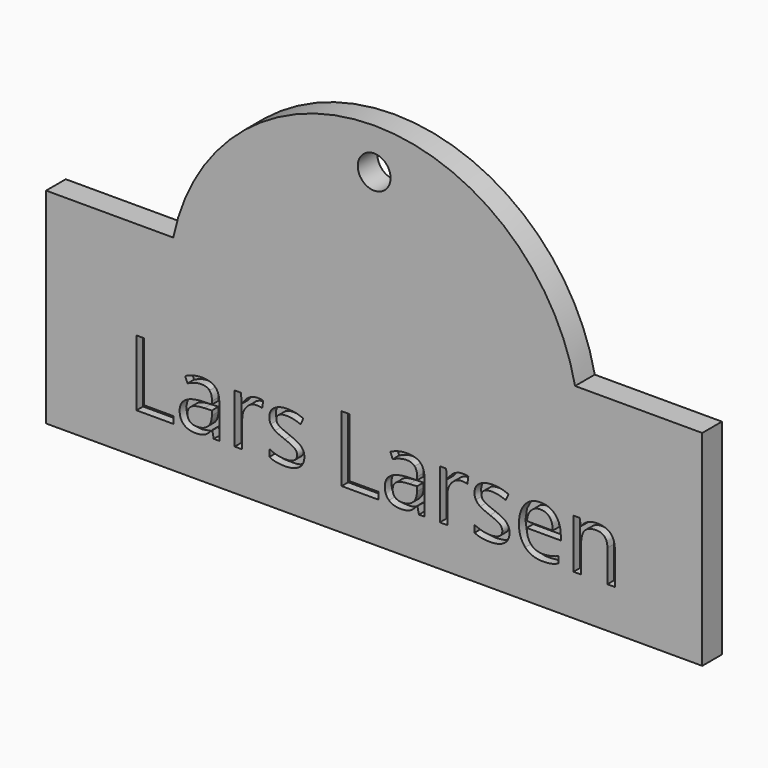
from build123d import *

# Parameters (mm, degrees)
F0_R         = 2
F1_DEPTH     = 3
F0_TEXT_SIZE = 11.2661289879
F2_DEPTH     = 2


# Not quite as in the source:
# - Text() gives the source's letters only with a copy of the font that has no kerning and outlines rounded to 1/6400 em; it was checked with that copy


with BuildPart() as f1:
    # F0 (on Front) → F1 (new body)
    with BuildSketch(Plane.XZ):
        with BuildLine():
            Line((-80.8457088497, 41.3709692657), (-96.3508114219, 41.3709692657))
            Line((-96.3508114219, 41.3709692657), (-96.3508114219, 16.3709692657))
            Line((-96.3508114219, 16.3709692657), (-16.3508114219, 16.3709692657))
            Line((-16.3508114219, 16.3709692657), (-16.3508114219, 41.3709692657))
            Line((-16.3508114219, 41.3709692657), (-31.855913994, 41.3709692657))
            ThreePointArc((-31.855913994, 41.3709692657), (-56.3508114219, 61.3709692657), (-80.8457088497, 41.3709692657))
        make_face()
        with BuildLine():
            Line((-75.2303791399, 21.3709692657), (-75.9081072118, 21.3709692657))
            Line((-75.9081072118, 21.3709692657), (-76.0894214752, 22.230011601))
            Line((-76.0894214752, 22.230011601), (-76.1334297916, 22.230011601))
            add(Edge.make_bspline(
                [(-76.1334297916, 22.230011601), (-76.5840749511, 21.6631844863), (-77.0320796116, 21.4616263974)],
                knots=[0, 0, 0, 1, 1, 1], degree=2))
            add(Edge.make_bspline(
                [(-77.0320796116, 21.4616263974), (-77.4800842721, 21.2600683085), (-78.1525313461, 21.2600683085)],
                knots=[0, 0, 0, 1, 1, 1], degree=2))
            add(Edge.make_bspline(
                [(-78.1525313461, 21.2600683085), (-79.0485406672, 21.2600683085), (-79.5572768043, 21.7230357966)],
                knots=[0, 0, 0, 1, 1, 1], degree=2))
            add(Edge.make_bspline(
                [(-79.5572768043, 21.7230357966), (-80.0660129414, 22.1860032847), (-80.0660129414, 23.0380042894)],
                knots=[0, 0, 0, 1, 1, 1], degree=2))
            add(Edge.make_bspline(
                [(-80.0660129414, 23.0380042894), (-80.0660129414, 24.8634692519), (-77.1456210678, 24.9514858847)],
                knots=[0, 0, 0, 1, 1, 1], degree=2))
            Line((-77.1456210678, 24.9514858847), (-76.1228677956, 24.9849322051))
            Line((-76.1228677956, 24.9849322051), (-76.1228677956, 25.3598830605))
            add(Edge.make_bspline(
                [(-76.1228677956, 25.3598830605), (-76.1228677956, 26.0692971202), (-76.4274053448, 26.4072809898)],
                knots=[0, 0, 0, 1, 1, 1], degree=2))
            add(Edge.make_bspline(
                [(-76.4274053448, 26.4072809898), (-76.731942894, 26.7452648595), (-77.404389968, 26.7452648595)],
                knots=[0, 0, 0, 1, 1, 1], degree=2))
            add(Edge.make_bspline(
                [(-77.404389968, 26.7452648595), (-78.1578123441, 26.7452648595), (-79.1083919774, 26.284057704)],
                knots=[0, 0, 0, 1, 1, 1], degree=2))
            Line((-79.1083919774, 26.284057704), (-79.3900452021, 26.9829097678))
            add(Edge.make_bspline(
                [(-79.3900452021, 26.9829097678), (-78.9446810406, 27.2240753414), (-78.4139407453, 27.3613812885)],
                knots=[0, 0, 0, 1, 1, 1], degree=2))
            add(Edge.make_bspline(
                [(-78.4139407453, 27.3613812885), (-77.88320045, 27.4986872355), (-77.3480593231, 27.4986872355)],
                knots=[0, 0, 0, 1, 1, 1], degree=2))
            add(Edge.make_bspline(
                [(-77.3480593231, 27.4986872355), (-76.2707357386, 27.4986872355), (-75.7505574392, 27.0207569199)],
                knots=[0, 0, 0, 1, 1, 1], degree=2))
            add(Edge.make_bspline(
                [(-75.7505574392, 27.0207569199), (-75.2303791399, 26.5428266042), (-75.2303791399, 25.4866270116)],
                knots=[0, 0, 0, 1, 1, 1], degree=2))
            Line((-75.2303791399, 25.4866270116), (-75.2303791399, 21.3709692657))
        make_face(mode=Mode.SUBTRACT)
        Polygon((-80.842319642, 21.3709692657), (-85.3258869126, 21.3709692657), (-85.3258869126, 29.4139291635), (-84.3911502732, 29.4139291635), (-84.3911502732, 22.2176892724), (-80.842319642, 22.2176892724), align=None, mode=Mode.SUBTRACT)
        with BuildLine():
            add(Edge.make_bspline(
                [(-71.639300525, 27.1915091873), (-71.165771041, 27.5110095641), (-70.5989439263, 27.5110095641)],
                knots=[0, 0, 0, 1, 1, 1], degree=2))
            add(Edge.make_bspline(
                [(-70.5989439263, 27.5110095641), (-70.1975880811, 27.5110095641), (-69.8789678706, 27.4441169232)],
                knots=[0, 0, 0, 1, 1, 1], degree=2))
            Line((-69.8789678706, 27.4441169232), (-70.0057118217, 26.5973969165))
            add(Edge.make_bspline(
                [(-70.0057118217, 26.5973969165), (-70.3789023445, 26.6801325512), (-70.6658365671, 26.6801325512)],
                knots=[0, 0, 0, 1, 1, 1], degree=2))
            add(Edge.make_bspline(
                [(-70.6658365671, 26.6801325512), (-71.3981349513, 26.6801325512), (-71.9174330844, 26.0860202804)],
                knots=[0, 0, 0, 1, 1, 1], degree=2))
            add(Edge.make_bspline(
                [(-71.9174330844, 26.0860202804), (-72.4367312174, 25.4919080096), (-72.4367312174, 24.6064606844)],
                knots=[0, 0, 0, 1, 1, 1], degree=2))
            Line((-72.4367312174, 24.6064606844), (-72.4367312174, 21.3709692657))
            Line((-72.4367312174, 21.3709692657), (-73.350343865, 21.3709692657))
            Line((-73.350343865, 21.3709692657), (-73.350343865, 27.4001086069))
            Line((-73.350343865, 27.4001086069), (-72.596921489, 27.4001086069))
            Line((-72.596921489, 27.4001086069), (-72.4913015297, 26.284057704))
            Line((-72.4913015297, 26.284057704), (-72.4472932133, 26.284057704))
            add(Edge.make_bspline(
                [(-72.4472932133, 26.284057704), (-72.112830009, 26.8720088106), (-71.639300525, 27.1915091873)],
                knots=[0, 0, 0, 1, 1, 1], degree=2))
        make_face(mode=Mode.SUBTRACT)
        with BuildLine():
            add(Edge.make_bspline(
                [(-65.2387309937, 24.0114682472), (-64.8620198057, 23.6153934), (-64.8620198057, 23.0151199649)],
                knots=[0, 0, 0, 1, 1, 1], degree=2))
            add(Edge.make_bspline(
                [(-64.8620198057, 23.0151199649), (-64.8620198057, 22.1736809561), (-65.4886982307, 21.7168746323)],
                knots=[0, 0, 0, 1, 1, 1], degree=2))
            add(Edge.make_bspline(
                [(-65.4886982307, 21.7168746323), (-66.1153766556, 21.2600683085), (-67.249030885, 21.2600683085)],
                knots=[0, 0, 0, 1, 1, 1], degree=2))
            add(Edge.make_bspline(
                [(-67.249030885, 21.2600683085), (-68.4478174226, 21.2600683085), (-69.1185041639, 21.6403001618)],
                knots=[0, 0, 0, 1, 1, 1], degree=2))
            Line((-69.1185041639, 21.6403001618), (-69.1185041639, 22.4870201686))
            add(Edge.make_bspline(
                [(-69.1185041639, 22.4870201686), (-68.6837019983, 22.2669785868), (-68.1864080235, 22.141114802)],
                knots=[0, 0, 0, 1, 1, 1], degree=2))
            add(Edge.make_bspline(
                [(-68.1864080235, 22.141114802), (-67.6891140486, 22.0152510172), (-67.2261465605, 22.0152510172)],
                knots=[0, 0, 0, 1, 1, 1], degree=2))
            add(Edge.make_bspline(
                [(-67.2261465605, 22.0152510172), (-66.5114515028, 22.0152510172), (-66.1268188179, 22.2432140959)],
                knots=[0, 0, 0, 1, 1, 1], degree=2))
            add(Edge.make_bspline(
                [(-66.1268188179, 22.2432140959), (-65.7421861329, 22.4711771747), (-65.7421861329, 22.9394256607)],
                knots=[0, 0, 0, 1, 1, 1], degree=2))
            add(Edge.make_bspline(
                [(-65.7421861329, 22.9394256607), (-65.7421861329, 23.2914921916), (-66.0467236821, 23.5414594285)],
                knots=[0, 0, 0, 1, 1, 1], degree=2))
            add(Edge.make_bspline(
                [(-66.0467236821, 23.5414594285), (-66.3512612313, 23.7914266654), (-67.2384688891, 24.1329312004)],
                knots=[0, 0, 0, 1, 1, 1], degree=2))
            add(Edge.make_bspline(
                [(-67.2384688891, 24.1329312004), (-68.0799078979, 24.4462704129), (-68.4346149277, 24.6803946559)],
                knots=[0, 0, 0, 1, 1, 1], degree=2))
            add(Edge.make_bspline(
                [(-68.4346149277, 24.6803946559), (-68.7893219576, 24.9145188989), (-68.962714724, 25.2111349512)],
                knots=[0, 0, 0, 1, 1, 1], degree=2))
            add(Edge.make_bspline(
                [(-68.962714724, 25.2111349512), (-69.1361074905, 25.5077510034), (-69.1361074905, 25.9196688446)],
                knots=[0, 0, 0, 1, 1, 1], degree=2))
            add(Edge.make_bspline(
                [(-69.1361074905, 25.9196688446), (-69.1361074905, 26.6572482267), (-68.5358340553, 27.0841288954)],
                knots=[0, 0, 0, 1, 1, 1], degree=2))
            add(Edge.make_bspline(
                [(-68.5358340553, 27.0841288954), (-67.9355606202, 27.5110095641), (-66.8916833562, 27.5110095641)],
                knots=[0, 0, 0, 1, 1, 1], degree=2))
            add(Edge.make_bspline(
                [(-66.8916833562, 27.5110095641), (-65.9182193983, 27.5110095641), (-64.9870034242, 27.1149347169)],
                knots=[0, 0, 0, 1, 1, 1], degree=2))
            Line((-64.9870034242, 27.1149347169), (-65.3126649652, 26.3720743367))
            add(Edge.make_bspline(
                [(-65.3126649652, 26.3720743367), (-66.2192362822, 26.7452648595), (-66.9568156644, 26.7452648595)],
                knots=[0, 0, 0, 1, 1, 1], degree=2))
            add(Edge.make_bspline(
                [(-66.9568156644, 26.7452648595), (-67.6063784138, 26.7452648595), (-67.9364407865, 26.5419464379)],
                knots=[0, 0, 0, 1, 1, 1], degree=2))
            add(Edge.make_bspline(
                [(-67.9364407865, 26.5419464379), (-68.2665031592, 26.3386280163), (-68.2665031592, 25.9812804875)],
                knots=[0, 0, 0, 1, 1, 1], degree=2))
            add(Edge.make_bspline(
                [(-68.2665031592, 25.9812804875), (-68.2665031592, 25.7383545812), (-68.1423997071, 25.56848248)],
                knots=[0, 0, 0, 1, 1, 1], degree=2))
            add(Edge.make_bspline(
                [(-68.1423997071, 25.56848248), (-68.018296255, 25.3986103789), (-67.7436843609, 25.2445812716)],
                knots=[0, 0, 0, 1, 1, 1], degree=2))
            add(Edge.make_bspline(
                [(-67.7436843609, 25.2445812716), (-67.4690724668, 25.0905521644), (-66.6874847683, 24.7983369437)],
                knots=[0, 0, 0, 1, 1, 1], degree=2))
            add(Edge.make_bspline(
                [(-66.6874847683, 24.7983369437), (-65.6154421818, 24.4075430945), (-65.2387309937, 24.0114682472)],
                knots=[0, 0, 0, 1, 1, 1], degree=2))
        make_face(mode=Mode.SUBTRACT)
        Polygon((-55.8279926235, 21.3709692657), (-60.3115598942, 21.3709692657), (-60.3115598942, 29.4139291635), (-59.3768232547, 29.4139291635), (-59.3768232547, 22.2176892724), (-55.8279926235, 22.2176892724), align=None, mode=Mode.SUBTRACT)
        with BuildLine():
            Line((-50.2160521214, 21.3709692657), (-50.8937801934, 21.3709692657))
            Line((-50.8937801934, 21.3709692657), (-51.0750944568, 22.230011601))
            Line((-51.0750944568, 22.230011601), (-51.1191027731, 22.230011601))
            add(Edge.make_bspline(
                [(-51.1191027731, 22.230011601), (-51.5697479326, 21.6631844863), (-52.0177525932, 21.4616263974)],
                knots=[0, 0, 0, 1, 1, 1], degree=2))
            add(Edge.make_bspline(
                [(-52.0177525932, 21.4616263974), (-52.4657572537, 21.2600683085), (-53.1382043277, 21.2600683085)],
                knots=[0, 0, 0, 1, 1, 1], degree=2))
            add(Edge.make_bspline(
                [(-53.1382043277, 21.2600683085), (-54.0342136487, 21.2600683085), (-54.5429497858, 21.7230357966)],
                knots=[0, 0, 0, 1, 1, 1], degree=2))
            add(Edge.make_bspline(
                [(-54.5429497858, 21.7230357966), (-55.051685923, 22.1860032847), (-55.051685923, 23.0380042894)],
                knots=[0, 0, 0, 1, 1, 1], degree=2))
            add(Edge.make_bspline(
                [(-55.051685923, 23.0380042894), (-55.051685923, 24.8634692519), (-52.1312940494, 24.9514858847)],
                knots=[0, 0, 0, 1, 1, 1], degree=2))
            Line((-52.1312940494, 24.9514858847), (-51.1085407772, 24.9849322051))
            Line((-51.1085407772, 24.9849322051), (-51.1085407772, 25.3598830605))
            add(Edge.make_bspline(
                [(-51.1085407772, 25.3598830605), (-51.1085407772, 26.0692971202), (-51.4130783264, 26.4072809898)],
                knots=[0, 0, 0, 1, 1, 1], degree=2))
            add(Edge.make_bspline(
                [(-51.4130783264, 26.4072809898), (-51.7176158756, 26.7452648595), (-52.3900629496, 26.7452648595)],
                knots=[0, 0, 0, 1, 1, 1], degree=2))
            add(Edge.make_bspline(
                [(-52.3900629496, 26.7452648595), (-53.1434853256, 26.7452648595), (-54.094064959, 26.284057704)],
                knots=[0, 0, 0, 1, 1, 1], degree=2))
            Line((-54.094064959, 26.284057704), (-54.3757181837, 26.9829097678))
            add(Edge.make_bspline(
                [(-54.3757181837, 26.9829097678), (-53.9303540221, 27.2240753414), (-53.3996137268, 27.3613812885)],
                knots=[0, 0, 0, 1, 1, 1], degree=2))
            add(Edge.make_bspline(
                [(-53.3996137268, 27.3613812885), (-52.8688734315, 27.4986872355), (-52.3337323046, 27.4986872355)],
                knots=[0, 0, 0, 1, 1, 1], degree=2))
            add(Edge.make_bspline(
                [(-52.3337323046, 27.4986872355), (-51.2564087202, 27.4986872355), (-50.7362304208, 27.0207569199)],
                knots=[0, 0, 0, 1, 1, 1], degree=2))
            add(Edge.make_bspline(
                [(-50.7362304208, 27.0207569199), (-50.2160521214, 26.5428266042), (-50.2160521214, 25.4866270116)],
                knots=[0, 0, 0, 1, 1, 1], degree=2))
            Line((-50.2160521214, 25.4866270116), (-50.2160521214, 21.3709692657))
        make_face(mode=Mode.SUBTRACT)
        with BuildLine():
            add(Edge.make_bspline(
                [(-46.6249735065, 27.1915091873), (-46.1514440225, 27.5110095641), (-45.5846169078, 27.5110095641)],
                knots=[0, 0, 0, 1, 1, 1], degree=2))
            add(Edge.make_bspline(
                [(-45.5846169078, 27.5110095641), (-45.1832610626, 27.5110095641), (-44.8646408522, 27.4441169232)],
                knots=[0, 0, 0, 1, 1, 1], degree=2))
            Line((-44.8646408522, 27.4441169232), (-44.9913848033, 26.5973969165))
            add(Edge.make_bspline(
                [(-44.9913848033, 26.5973969165), (-45.364575326, 26.6801325512), (-45.6515095487, 26.6801325512)],
                knots=[0, 0, 0, 1, 1, 1], degree=2))
            add(Edge.make_bspline(
                [(-45.6515095487, 26.6801325512), (-46.3838079329, 26.6801325512), (-46.9031060659, 26.0860202804)],
                knots=[0, 0, 0, 1, 1, 1], degree=2))
            add(Edge.make_bspline(
                [(-46.9031060659, 26.0860202804), (-47.422404199, 25.4919080096), (-47.422404199, 24.6064606844)],
                knots=[0, 0, 0, 1, 1, 1], degree=2))
            Line((-47.422404199, 24.6064606844), (-47.422404199, 21.3709692657))
            Line((-47.422404199, 21.3709692657), (-48.3360168466, 21.3709692657))
            Line((-48.3360168466, 21.3709692657), (-48.3360168466, 27.4001086069))
            Line((-48.3360168466, 27.4001086069), (-47.5825944705, 27.4001086069))
            Line((-47.5825944705, 27.4001086069), (-47.4769745112, 26.284057704))
            Line((-47.4769745112, 26.284057704), (-47.4329661949, 26.284057704))
            add(Edge.make_bspline(
                [(-47.4329661949, 26.284057704), (-47.0985029906, 26.8720088106), (-46.6249735065, 27.1915091873)],
                knots=[0, 0, 0, 1, 1, 1], degree=2))
        make_face(mode=Mode.SUBTRACT)
        with BuildLine():
            add(Edge.make_bspline(
                [(-40.2244039753, 24.0114682472), (-39.8476927872, 23.6153934), (-39.8476927872, 23.0151199649)],
                knots=[0, 0, 0, 1, 1, 1], degree=2))
            add(Edge.make_bspline(
                [(-39.8476927872, 23.0151199649), (-39.8476927872, 22.1736809561), (-40.4743712122, 21.7168746323)],
                knots=[0, 0, 0, 1, 1, 1], degree=2))
            add(Edge.make_bspline(
                [(-40.4743712122, 21.7168746323), (-41.1010496372, 21.2600683085), (-42.2347038666, 21.2600683085)],
                knots=[0, 0, 0, 1, 1, 1], degree=2))
            add(Edge.make_bspline(
                [(-42.2347038666, 21.2600683085), (-43.4334904042, 21.2600683085), (-44.1041771455, 21.6403001618)],
                knots=[0, 0, 0, 1, 1, 1], degree=2))
            Line((-44.1041771455, 21.6403001618), (-44.1041771455, 22.4870201686))
            add(Edge.make_bspline(
                [(-44.1041771455, 22.4870201686), (-43.6693749799, 22.2669785868), (-43.172081005, 22.141114802)],
                knots=[0, 0, 0, 1, 1, 1], degree=2))
            add(Edge.make_bspline(
                [(-43.172081005, 22.141114802), (-42.6747870302, 22.0152510172), (-42.2118195421, 22.0152510172)],
                knots=[0, 0, 0, 1, 1, 1], degree=2))
            add(Edge.make_bspline(
                [(-42.2118195421, 22.0152510172), (-41.4971244844, 22.0152510172), (-41.1124917994, 22.2432140959)],
                knots=[0, 0, 0, 1, 1, 1], degree=2))
            add(Edge.make_bspline(
                [(-41.1124917994, 22.2432140959), (-40.7278591144, 22.4711771747), (-40.7278591144, 22.9394256607)],
                knots=[0, 0, 0, 1, 1, 1], degree=2))
            add(Edge.make_bspline(
                [(-40.7278591144, 22.9394256607), (-40.7278591144, 23.2914921916), (-41.0323966636, 23.5414594285)],
                knots=[0, 0, 0, 1, 1, 1], degree=2))
            add(Edge.make_bspline(
                [(-41.0323966636, 23.5414594285), (-41.3369342128, 23.7914266654), (-42.2241418706, 24.1329312004)],
                knots=[0, 0, 0, 1, 1, 1], degree=2))
            add(Edge.make_bspline(
                [(-42.2241418706, 24.1329312004), (-43.0655808794, 24.4462704129), (-43.4202879093, 24.6803946559)],
                knots=[0, 0, 0, 1, 1, 1], degree=2))
            add(Edge.make_bspline(
                [(-43.4202879093, 24.6803946559), (-43.7749949391, 24.9145188989), (-43.9483877056, 25.2111349512)],
                knots=[0, 0, 0, 1, 1, 1], degree=2))
            add(Edge.make_bspline(
                [(-43.9483877056, 25.2111349512), (-44.121780472, 25.5077510034), (-44.121780472, 25.9196688446)],
                knots=[0, 0, 0, 1, 1, 1], degree=2))
            add(Edge.make_bspline(
                [(-44.121780472, 25.9196688446), (-44.121780472, 26.6572482267), (-43.5215070369, 27.0841288954)],
                knots=[0, 0, 0, 1, 1, 1], degree=2))
            add(Edge.make_bspline(
                [(-43.5215070369, 27.0841288954), (-42.9212336018, 27.5110095641), (-41.8773563377, 27.5110095641)],
                knots=[0, 0, 0, 1, 1, 1], degree=2))
            add(Edge.make_bspline(
                [(-41.8773563377, 27.5110095641), (-40.9038923799, 27.5110095641), (-39.9726764057, 27.1149347169)],
                knots=[0, 0, 0, 1, 1, 1], degree=2))
            Line((-39.9726764057, 27.1149347169), (-40.2983379468, 26.3720743367))
            add(Edge.make_bspline(
                [(-40.2983379468, 26.3720743367), (-41.2049092638, 26.7452648595), (-41.9424886459, 26.7452648595)],
                knots=[0, 0, 0, 1, 1, 1], degree=2))
            add(Edge.make_bspline(
                [(-41.9424886459, 26.7452648595), (-42.5920513954, 26.7452648595), (-42.9221137681, 26.5419464379)],
                knots=[0, 0, 0, 1, 1, 1], degree=2))
            add(Edge.make_bspline(
                [(-42.9221137681, 26.5419464379), (-43.2521761408, 26.3386280163), (-43.2521761408, 25.9812804875)],
                knots=[0, 0, 0, 1, 1, 1], degree=2))
            add(Edge.make_bspline(
                [(-43.2521761408, 25.9812804875), (-43.2521761408, 25.7383545812), (-43.1280726886, 25.56848248)],
                knots=[0, 0, 0, 1, 1, 1], degree=2))
            add(Edge.make_bspline(
                [(-43.1280726886, 25.56848248), (-43.0039692365, 25.3986103789), (-42.7293573424, 25.2445812716)],
                knots=[0, 0, 0, 1, 1, 1], degree=2))
            add(Edge.make_bspline(
                [(-42.7293573424, 25.2445812716), (-42.4547454484, 25.0905521644), (-41.6731577498, 24.7983369437)],
                knots=[0, 0, 0, 1, 1, 1], degree=2))
            add(Edge.make_bspline(
                [(-41.6731577498, 24.7983369437), (-40.6011151633, 24.4075430945), (-40.2244039753, 24.0114682472)],
                knots=[0, 0, 0, 1, 1, 1], degree=2))
        make_face(mode=Mode.SUBTRACT)
        with BuildLine():
            add(Edge.make_bspline(
                [(-34.7726537447, 21.3516056065), (-35.203935245, 21.2600683085), (-35.8147706761, 21.2600683085)],
                knots=[0, 0, 0, 1, 1, 1], degree=2))
            add(Edge.make_bspline(
                [(-35.8147706761, 21.2600683085), (-37.1508631608, 21.2600683085), (-37.9245293624, 22.0751023274)],
                knots=[0, 0, 0, 1, 1, 1], degree=2))
            add(Edge.make_bspline(
                [(-37.9245293624, 22.0751023274), (-38.698195564, 22.8901363464), (-38.698195564, 24.3353694556)],
                knots=[0, 0, 0, 1, 1, 1], degree=2))
            add(Edge.make_bspline(
                [(-38.698195564, 24.3353694556), (-38.698195564, 25.7946852261), (-37.979979841, 26.6528473951)],
                knots=[0, 0, 0, 1, 1, 1], degree=2))
            add(Edge.make_bspline(
                [(-37.979979841, 26.6528473951), (-37.261764118, 27.5110095641), (-36.0506552518, 27.5110095641)],
                knots=[0, 0, 0, 1, 1, 1], degree=2))
            add(Edge.make_bspline(
                [(-36.0506552518, 27.5110095641), (-34.918761355, 27.5110095641), (-34.2586366097, 26.765508685)],
                knots=[0, 0, 0, 1, 1, 1], degree=2))
            add(Edge.make_bspline(
                [(-34.2586366097, 26.765508685), (-33.5985118643, 26.0200078059), (-33.5985118643, 24.7983369437)],
                knots=[0, 0, 0, 1, 1, 1], degree=2))
            Line((-33.5985118643, 24.7983369437), (-33.5985118643, 24.2209478331))
            Line((-33.5985118643, 24.2209478331), (-37.7511365959, 24.2209478331))
            add(Edge.make_bspline(
                [(-37.7511365959, 24.2209478331), (-37.7229712734, 23.1594672425), (-37.2142351363, 22.609363288)],
                knots=[0, 0, 0, 1, 1, 1], degree=2))
            add(Edge.make_bspline(
                [(-37.2142351363, 22.609363288), (-36.7054989992, 22.0592593336), (-35.7813243557, 22.0592593336)],
                knots=[0, 0, 0, 1, 1, 1], degree=2))
            add(Edge.make_bspline(
                [(-35.7813243557, 22.0592593336), (-34.8078603978, 22.0592593336), (-33.8572807645, 22.4658961767)],
                knots=[0, 0, 0, 1, 1, 1], degree=2))
            Line((-33.8572807645, 22.4658961767), (-33.8572807645, 21.6508621577))
            add(Edge.make_bspline(
                [(-33.8572807645, 21.6508621577), (-34.3413722444, 21.4431429045), (-34.7726537447, 21.3516056065)],
                knots=[0, 0, 0, 1, 1, 1], degree=2))
        make_face(mode=Mode.SUBTRACT)
        with BuildLine():
            Line((-27.0007850757, 21.3709692657), (-27.9143977233, 21.3709692657))
            Line((-27.9143977233, 21.3709692657), (-27.9143977233, 25.2718664278))
            add(Edge.make_bspline(
                [(-27.9143977233, 25.2718664278), (-27.9143977233, 26.0076854773), (-28.249741094, 26.3711941704)],
                knots=[0, 0, 0, 1, 1, 1], degree=2))
            add(Edge.make_bspline(
                [(-28.249741094, 26.3711941704), (-28.5850844647, 26.7347028635), (-29.301539855, 26.7347028635)],
                knots=[0, 0, 0, 1, 1, 1], degree=2))
            add(Edge.make_bspline(
                [(-29.301539855, 26.7347028635), (-30.2468384904, 26.7347028635), (-30.686921654, 26.2233262274)],
                knots=[0, 0, 0, 1, 1, 1], degree=2))
            add(Edge.make_bspline(
                [(-30.686921654, 26.2233262274), (-31.1270048176, 25.7119495914), (-31.1270048176, 24.5342870456)],
                knots=[0, 0, 0, 1, 1, 1], degree=2))
            Line((-31.1270048176, 24.5342870456), (-31.1270048176, 21.3709692657))
            Line((-31.1270048176, 21.3709692657), (-32.0406174652, 21.3709692657))
            Line((-32.0406174652, 21.3709692657), (-32.0406174652, 27.4001086069))
            Line((-32.0406174652, 27.4001086069), (-31.297757085, 27.4001086069))
            Line((-31.297757085, 27.4001086069), (-31.1498891421, 26.574512592))
            Line((-31.1498891421, 26.574512592), (-31.1058808257, 26.574512592))
            add(Edge.make_bspline(
                [(-31.1058808257, 26.574512592), (-30.824227601, 27.0198767535), (-30.3181319629, 27.2654431588)],
                knots=[0, 0, 0, 1, 1, 1], degree=2))
            add(Edge.make_bspline(
                [(-30.3181319629, 27.2654431588), (-29.8120363247, 27.5110095641), (-29.1906388978, 27.5110095641)],
                knots=[0, 0, 0, 1, 1, 1], degree=2))
            add(Edge.make_bspline(
                [(-29.1906388978, 27.5110095641), (-28.1009929847, 27.5110095641), (-27.5508890302, 26.9855502668)],
                knots=[0, 0, 0, 1, 1, 1], degree=2))
            add(Edge.make_bspline(
                [(-27.5508890302, 26.9855502668), (-27.0007850757, 26.4600909695), (-27.0007850757, 25.3035524155)],
                knots=[0, 0, 0, 1, 1, 1], degree=2))
            Line((-27.0007850757, 25.3035524155), (-27.0007850757, 21.3709692657))
        make_face(mode=Mode.SUBTRACT)
        with Locations((-56.3508114219, 56.3709692657)):
            Circle(F0_R, mode=Mode.SUBTRACT)
    extrude(amount=F1_DEPTH)


with BuildPart() as f1b:
    # F0 (on Front) → F1, piece 2 (new body)
    with BuildSketch(Plane.XZ):
        with BuildLine():
            add(Edge.make_bspline(
                [(-78.8091354262, 22.2731397511), (-78.509878875, 22.0152510172), (-77.9712170827, 22.0152510172)],
                knots=[0, 0, 0, 1, 1, 1], degree=2))
            add(Edge.make_bspline(
                [(-77.9712170827, 22.0152510172), (-77.1174557454, 22.0152510172), (-76.6307237664, 22.4826193369)],
                knots=[0, 0, 0, 1, 1, 1], degree=2))
            add(Edge.make_bspline(
                [(-76.6307237664, 22.4826193369), (-76.1439917875, 22.9499876567), (-76.1439917875, 23.7914266654)],
                knots=[0, 0, 0, 1, 1, 1], degree=2))
            Line((-76.1439917875, 23.7914266654), (-76.1439917875, 24.3353694556))
            Line((-76.1439917875, 24.3353694556), (-77.0576044351, 24.2984024699))
            add(Edge.make_bspline(
                [(-77.0576044351, 24.2984024699), (-78.1472503482, 24.2596751515), (-78.6278211628, 23.9595384339)],
                knots=[0, 0, 0, 1, 1, 1], degree=2))
            add(Edge.make_bspline(
                [(-78.6278211628, 23.9595384339), (-79.1083919774, 23.6594017164), (-79.1083919774, 23.0274422935)],
                knots=[0, 0, 0, 1, 1, 1], degree=2))
            add(Edge.make_bspline(
                [(-79.1083919774, 23.0274422935), (-79.1083919774, 22.5310284849), (-78.8091354262, 22.2731397511)],
                knots=[0, 0, 0, 1, 1, 1], degree=2))
        make_face()
    extrude(amount=F1_DEPTH)


with BuildPart() as f1c:
    # F0 (on Front) → F1, piece 3 (new body)
    with BuildSketch(Plane.XZ):
        with BuildLine():
            add(Edge.make_bspline(
                [(-53.7948084077, 22.2731397511), (-53.4955518565, 22.0152510172), (-52.9568900643, 22.0152510172)],
                knots=[0, 0, 0, 1, 1, 1], degree=2))
            add(Edge.make_bspline(
                [(-52.9568900643, 22.0152510172), (-52.1031287269, 22.0152510172), (-51.616396748, 22.4826193369)],
                knots=[0, 0, 0, 1, 1, 1], degree=2))
            add(Edge.make_bspline(
                [(-51.616396748, 22.4826193369), (-51.129664769, 22.9499876567), (-51.129664769, 23.7914266654)],
                knots=[0, 0, 0, 1, 1, 1], degree=2))
            Line((-51.129664769, 23.7914266654), (-51.129664769, 24.3353694556))
            Line((-51.129664769, 24.3353694556), (-52.0432774167, 24.2984024699))
            add(Edge.make_bspline(
                [(-52.0432774167, 24.2984024699), (-53.1329233297, 24.2596751515), (-53.6134941443, 23.9595384339)],
                knots=[0, 0, 0, 1, 1, 1], degree=2))
            add(Edge.make_bspline(
                [(-53.6134941443, 23.9595384339), (-54.094064959, 23.6594017164), (-54.094064959, 23.0274422935)],
                knots=[0, 0, 0, 1, 1, 1], degree=2))
            add(Edge.make_bspline(
                [(-54.094064959, 23.0274422935), (-54.094064959, 22.5310284849), (-53.7948084077, 22.2731397511)],
                knots=[0, 0, 0, 1, 1, 1], degree=2))
        make_face()
    extrude(amount=F1_DEPTH)


with BuildPart() as f1d:
    # F0 (on Front) → F1, piece 4 (new body)
    with BuildSketch(Plane.XZ):
        with BuildLine():
            add(Edge.make_bspline(
                [(-34.9618895051, 26.2858180367), (-35.3465221901, 26.7452648595), (-36.0629775804, 26.7452648595)],
                knots=[0, 0, 0, 1, 1, 1], degree=2))
            add(Edge.make_bspline(
                [(-36.0629775804, 26.7452648595), (-36.788234634, 26.7452648595), (-37.2203963006, 26.2726155418)],
                knots=[0, 0, 0, 1, 1, 1], degree=2))
            add(Edge.make_bspline(
                [(-37.2203963006, 26.2726155418), (-37.6525579673, 25.7999662241), (-37.7300126041, 24.9638082132)],
                knots=[0, 0, 0, 1, 1, 1], degree=2))
            Line((-37.7300126041, 24.9638082132), (-34.5772568201, 24.9638082132))
            add(Edge.make_bspline(
                [(-34.5772568201, 24.9638082132), (-34.5772568201, 25.8263712139), (-34.9618895051, 26.2858180367)],
                knots=[0, 0, 0, 1, 1, 1], degree=2))
        make_face()
    extrude(amount=F1_DEPTH)


with BuildPart() as f2:
    # F0 (on Front) → F2 (new body)
    with BuildSketch(Plane.XZ):
        with Locations((-86.4313758196, 21.3709692657)):
            Text('Lars Larsen', F0_TEXT_SIZE, font='Open Sans', text_align=(TextAlign.LEFT, TextAlign.BOTTOM))
    extrude(amount=F2_DEPTH)


solid = Compound([f1.part, f1b.part, f1c.part, f1d.part, f2.part])
